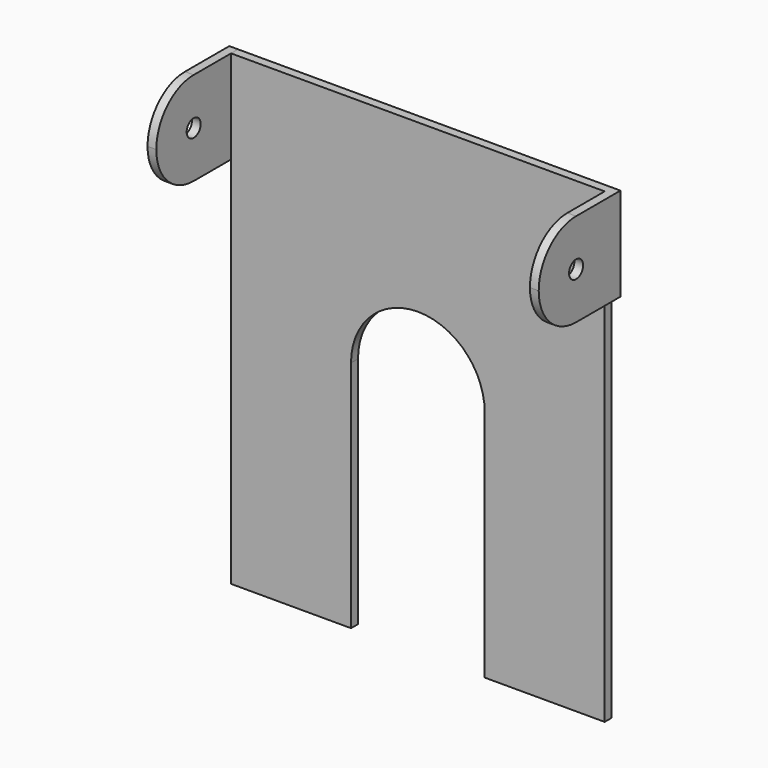
from build123d import *

# Parameters (mm, degrees)
F1_DEPTH = 4.7625
F2_W     = 4.7625
F2_H     = 50.8
F3_DEPTH = 55.5625
F4_R     = 4.7625
F5_DEPTH = 4.7625
F6_R     = 25.39999


# Not quite as in the source:
# - a fillet or chamfer is up to 0.001 mm smaller than in the source, because OpenCascade refuses the exact size


with BuildPart() as f1:
    # F0 (on Front) → F1 (new body)
    with BuildSketch(Plane.XZ):
        with BuildLine():
            Line((-101.6, 127), (-101.6, -127))
            Line((-101.6, -127), (-36.3640275955, -127))
            Line((-36.3640275955, -127), (-36.3640275955, 0))
            ThreePointArc((-36.3640275955, 0), (-25.713250504, 25.713250504), (0, 36.3640275955))
            Line((0, 36.3640275955), (0, 127))
            Line((0, 127), (-101.6, 127))
        make_face()
    extrude(amount=F1_DEPTH)



with BuildPart() as f3:
    # F2 (on Front) → F3 (new body)
    with BuildSketch(Plane.XZ):
        with Locations((-103.98125, 101.6)):
            Rectangle(F2_W, F2_H)
    extrude(amount=F3_DEPTH)

    # F4 (on face) → F5 (cut, through all)
    with BuildSketch(Plane(origin=(-106.3625, 0, 0), x_dir=(0, -1, 0), z_dir=(-1, 0, 0))):
        with Locations((30.1625, 101.6)):
            Circle(F4_R)
    extrude(amount=-F5_DEPTH, mode=Mode.SUBTRACT)

    # F6 (radius 25.4 in the source; OpenCascade refuses exactly that, so slightly less here)
    f6_edges = [f3.edges().sort_by_distance(p)[0] for p in [
        (-103.98125, -55.5625, 127),
        (-103.98125, -55.5625, 76.2),
    ]]
    fillet(f6_edges, radius=F6_R)


with BuildPart() as f1_1:
    add(f1.part)
    # F7: F3, F1 across plane
    add(f3.part.mirror(Plane.YZ))
    add(f1.part.mirror(Plane.YZ))


solid = Compound([f3.part, f1_1.part])
